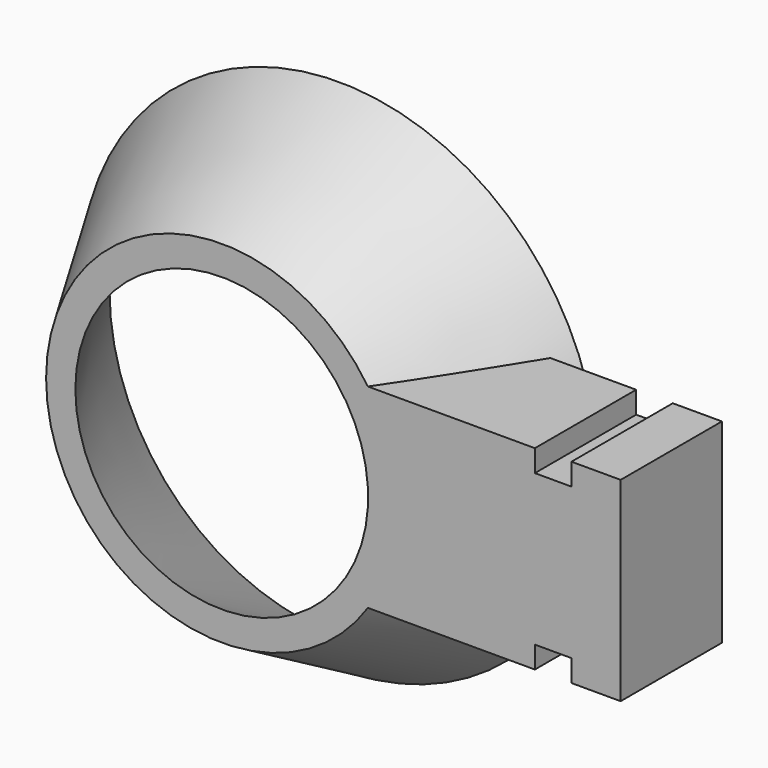
from build123d import *

# Parameters (mm, degrees)
F3_W     = 8.786383085
F3_H     = 13.5255949572
F5_DEPTH = 10.16
F6_W     = 2.54
F6_H     = 8.786383085
F7_DEPTH = 1.524


# Not quite as in the source:
# - a pattern or mirror of a feature is missing from the dataset's text; its kind, count and spacing are read off the source's solid


with BuildPart() as f1:
    # F0 (on Top) → F1 (revolve)
    with BuildSketch(Plane.XY):
        Polygon((-12.192, 0), (-10.16, 0), (-15.9150013827, 10.16), (-17.9470013827, 10.16), align=None)
    revolve(axis=Axis((0, 4.3423168827, 0), (0, -1, 0)))

    # F3 (on offset) → F4 (join, up to the next surface of F1)
    with BuildSketch(Plane.YZ.offset(17.526)):
        with Locations((4.3931915425, 0)):
            Rectangle(F3_W, F3_H)
    extrude(until=Until.NEXT, dir=(-1, 0, 0))

    # F5 (add): a face of the model
    f5_faces = [f1.faces().sort_by_distance(p)[0] for p in [
        (17.526, 4.3931915425, 0),
    ]]
    extrude(f5_faces, amount=F5_DEPTH)

    # F6 (on face) → F7 (cut)
    with BuildSketch(Plane.XY.offset(6.7627974786)):
        with Locations((23.0034508117, 4.3931915425)):
            Rectangle(F6_W, F6_H)
    f7 = extrude(amount=-F7_DEPTH, mode=Mode.SUBTRACT)

    # F7_copies: F7 across plane
    add(f7.mirror(Plane(origin=(0, 0, 0), x_dir=(-1, 0, 0), z_dir=(0, 0, -1))), mode=Mode.SUBTRACT)


solid = f1.part
